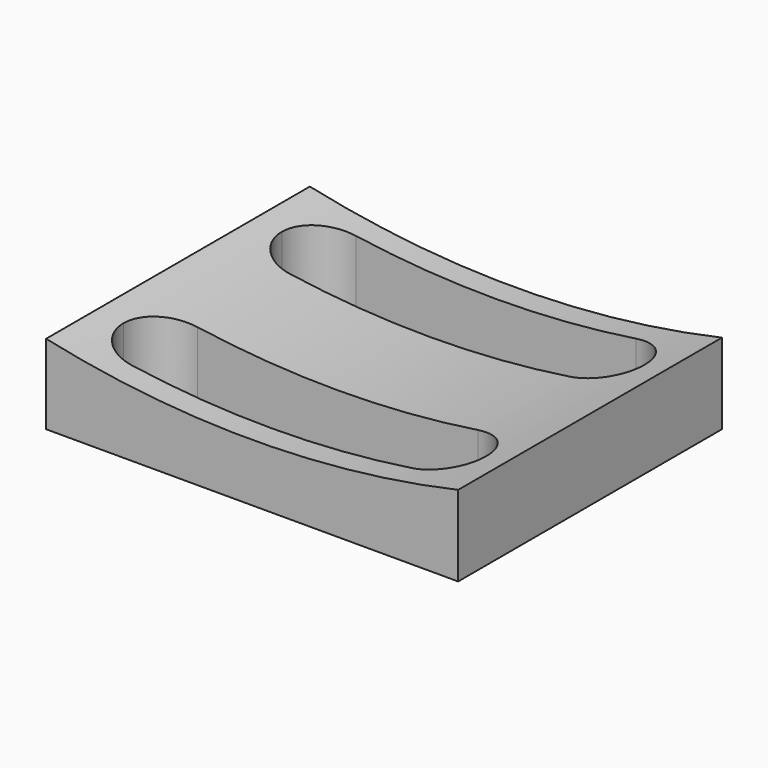
from build123d import *

# Parameters (mm, degrees)
F0_W     = 50
F0_H     = 40
F1_DEPTH = 10
F3_DEPTH = 40
F5_W     = 44
F5_H     = 10
F6_DEPTH = 18
F7_R     = 4.99999


# Not quite as in the source:
# - a fillet or chamfer is up to 0.001 mm smaller than in the source, because OpenCascade refuses the exact size


with BuildPart() as f1:
    # F0 (on Top) → F1 (new body)
    with BuildSketch(Plane.XY):
        Rectangle(F0_W, F0_H)
    extrude(amount=F1_DEPTH)

    # F2 (on face) → F3 (cut)
    with BuildSketch(Plane.XZ.offset(20)):
        with BuildLine():
            Line((-25, 10), (-25, 9.6663655309))
            ThreePointArc((-25, 9.6663655309), (0.0065046461, 7.0000153387), (25, 9.7856728837))
            Line((25, 9.7856728837), (25, 10))
            Line((25, 10), (-25, 10))
        make_face()
    extrude(amount=-F3_DEPTH, mode=Mode.SUBTRACT)

    # F5 (on offset) → F6 (cut)
    with BuildSketch(Plane.XY.offset(10)):
        with Locations((0, 12)):
            Rectangle(F5_W, F5_H)
        with Locations((0, -12)):
            Rectangle(F5_W, F5_H)
    extrude(amount=-F6_DEPTH, mode=Mode.SUBTRACT)

    # F7 (radius 5 in the source; OpenCascade refuses exactly that, so slightly less here)
    f7_edges = [f1.edges().sort_by_distance(p)[0] for p in [
        (-22, 17, 4.52656),
        (22, 17, 4.578769),
        (-22, -7, 4.52656),
        (22, -7, 4.578769),
        (-22, -17, 4.52656),
        (22, -17, 4.578769),
        (22, 7, 4.578769),
        (-22, 7, 4.52656),
    ]]
    fillet(f7_edges, radius=F7_R)


solid = f1.part
